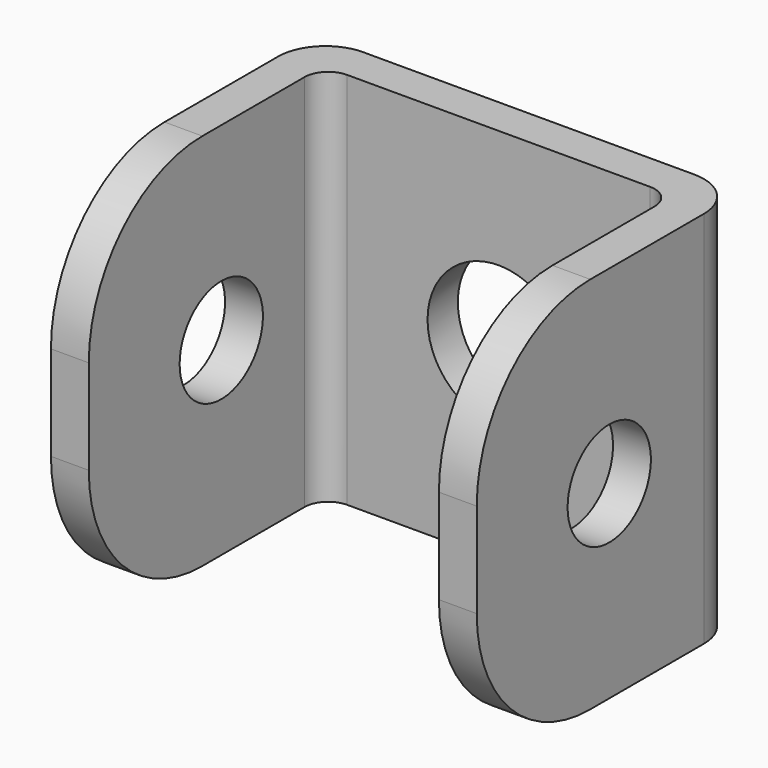
from build123d import *

# Parameters (mm, degrees)
F0_W     = 90
F0_H     = 80
F1_DEPTH = 70
F2_T     = -8
F3_R     = 5
F4_R     = 10
F5_R     = 30
F7_D     = 30
F9_D     = 22


with BuildPart() as f1:
    # F0 (on Front) → F1 (new body)
    with BuildSketch(Plane.XZ):
        Rectangle(F0_W, F0_H)
    extrude(amount=F1_DEPTH)

    # F2
    f2_openings = [f1.faces().sort_by_distance(p)[0] for p in [
        (0, -70, 0),
        (0, -35, 40),
        (0, -35, -40),
    ]]
    offset(amount=F2_T, openings=f2_openings)

    # F3
    f3_edges = [f1.edges().sort_by_distance(p)[0] for p in [
        (-37, -8, 0),
        (37, -8, 0),
    ]]
    fillet(f3_edges, radius=F3_R)

    # F4
    f4_edges = [f1.edges().sort_by_distance(p)[0] for p in [
        (-45, 0, 0),
        (45, 0, 0),
    ]]
    fillet(f4_edges, radius=F4_R)

    # F5
    f5_edges = [f1.edges().sort_by_distance(p)[0] for p in [
        (41, -70, 40),
        (-41, -70, 40),
        (41, -70, -40),
        (-41, -70, -40),
    ]]
    fillet(f5_edges, radius=F5_R)

    # F7 (through all)
    with Locations(Plane.XZ.offset(8)):
        with Locations((0, 0)):
            Hole(F7_D / 2)

    # F9 (through all)
    with Locations(Plane.YZ.offset(45)):
        with Locations((-35, 0)):
            Hole(F9_D / 2)


solid = f1.part
